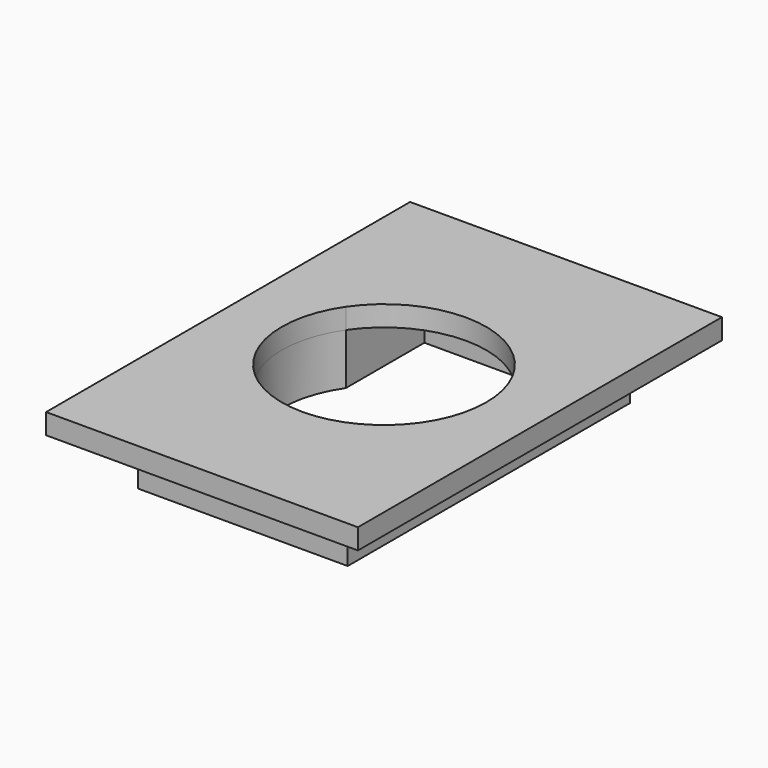
from build123d import *
from build123d import SkipClean  # not in build123d's __all__

# Parameters (mm, degrees)
F0_W     = 30.5
F0_H     = 44.5
F0_W_2   = 20.5
F0_H_2   = 34.5
F1_DEPTH = 2
F2_DEPTH = 5


with BuildPart() as f1:
    # F0 (on Top) → F1 (new body)
    with BuildSketch(Plane.XY):
        Rectangle(F0_W, F0_H)
        Rectangle(F0_W_2, F0_H_2, mode=Mode.SUBTRACT)
        Rectangle(F0_W_2, F0_H_2)
        with BuildLine():
            ThreePointArc((8.25, 5.6513272777), (9.5524865873, 2.9580398915), (10, 0))
            ThreePointArc((10, 0), (9.5524865873, -2.9580398915), (8.25, -5.6513272777))
            Line((8.25, -5.6513272777), (8.25, -15.25))
            Line((8.25, -15.25), (-8.25, -15.25))
            Line((-8.25, -15.25), (-8.25, -5.6513272777))
            ThreePointArc((-8.25, -5.6513272777), (-10, 0), (-8.25, 5.6513272777))
            Line((-8.25, 5.6513272777), (-8.25, 15.25))
            Line((-8.25, 15.25), (8.25, 15.25))
            Line((8.25, 15.25), (8.25, 5.6513272777))
        make_face(mode=Mode.SUBTRACT)
        with BuildLine():
            ThreePointArc((-8.25, 5.6513272777), (0, 10), (8.25, 5.6513272777))
            Line((8.25, 5.6513272777), (8.25, 15.25))
            Line((8.25, 15.25), (-8.25, 15.25))
            Line((-8.25, 15.25), (-8.25, 5.6513272777))
        make_face()
        with BuildLine():
            Line((8.25, -15.25), (8.25, -5.6513272777))
            ThreePointArc((8.25, -5.6513272777), (0, -10), (-8.25, -5.6513272777))
            Line((-8.25, -5.6513272777), (-8.25, -15.25))
            Line((-8.25, -15.25), (8.25, -15.25))
        make_face()
    extrude(amount=F1_DEPTH)

    # F0 (on Top) → F2 (join)
    with BuildSketch(Plane.XY):
        Rectangle(F0_W_2, F0_H_2)
        with BuildLine():
            ThreePointArc((8.25, 5.6513272777), (9.5524865873, 2.9580398915), (10, 0))
            ThreePointArc((10, 0), (9.5524865873, -2.9580398915), (8.25, -5.6513272777))
            Line((8.25, -5.6513272777), (8.25, -15.25))
            Line((8.25, -15.25), (-8.25, -15.25))
            Line((-8.25, -15.25), (-8.25, -5.6513272777))
            ThreePointArc((-8.25, -5.6513272777), (-10, 0), (-8.25, 5.6513272777))
            Line((-8.25, 5.6513272777), (-8.25, 15.25))
            Line((-8.25, 15.25), (8.25, 15.25))
            Line((8.25, 15.25), (8.25, 5.6513272777))
        make_face(mode=Mode.SUBTRACT)
    with SkipClean():  # cleaning this boolean's faces spoils the solid; the shape is the same uncleaned
        extrude(amount=-F2_DEPTH)


solid = f1.part
